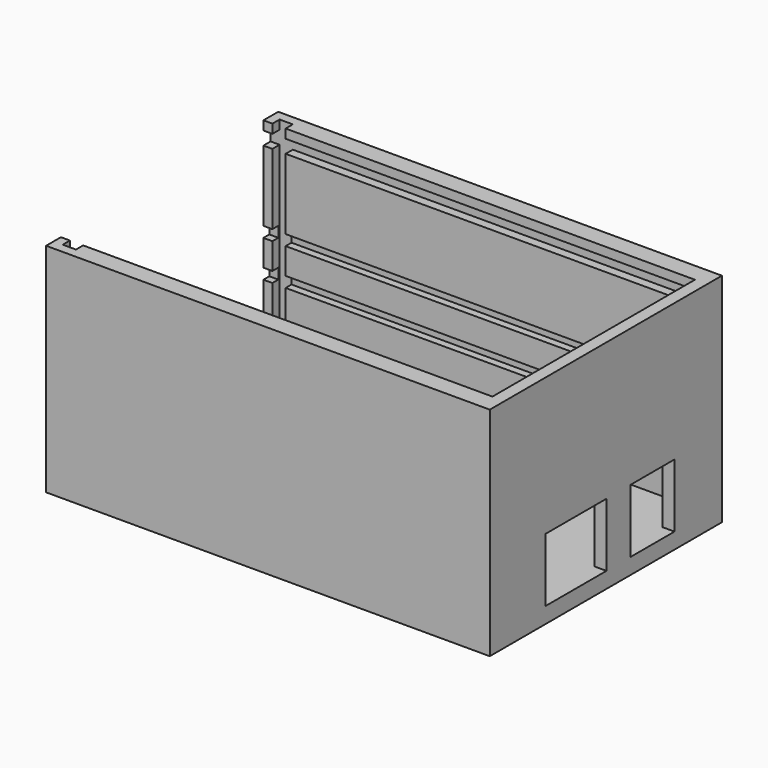
from build123d import *

# Parameters (mm, degrees)
F2_DEPTH  = 41
F1_W      = 1.7
F1_H      = 47.8
F1_W_2    = 77.3
F3_DEPTH  = 3
F1_W_3    = 2.5
F1_H_2    = 1.7
F4_DEPTH  = 1.5
F5_W      = 14.41
F5_H      = 12
F5_W_2    = 10.4
F6_DEPTH  = 3
F7_W      = 1.4
F7_H      = 2
F8_DEPTH  = 81
F9_W      = 1.7
F9_H      = 2.5
F10_DEPTH = 83
F11_W     = 47.8
F11_H     = 2.5
F12_DEPTH = 1.5


with BuildPart() as f2:
    # F1 (on Top) → F2 (new body)
    with BuildSketch(Plane.XY):
        Polygon((-43, 27.4), (-43, 23.9), (-41.3, 23.9), (-41.3, 25.6), (-38.8, 25.6), (-38.8, 23.9), (38.5, 23.9), (38.5, -23.9), (-38.8, -23.9), (-38.8, -25.6), (-41.3, -25.6), (-41.3, -23.9), (-43, -23.9), (-43, -27.4), (40.8, -27.4), (40.8, 27.4), align=None)
    extrude(amount=F2_DEPTH)

    # F1 (on Top) → F3 (join)
    with BuildSketch(Plane.XY):
        with Locations((-42.15, 0)):
            Rectangle(F1_W, F1_H)
        with Locations((-0.15, 0)):
            Rectangle(F1_W_2, F1_H)
    extrude(amount=F3_DEPTH)

    # F1 (on Top) → F4 (join)
    with BuildSketch(Plane.XY):
        with Locations((-40.05, -24.75)):
            Rectangle(F1_W_3, F1_H_2)
        with Locations((-40.05, 0)):
            Rectangle(F1_W_3, F1_H)
        with Locations((-40.05, 24.75)):
            Rectangle(F1_W_3, F1_H_2)
    extrude(amount=F4_DEPTH)

    # F5 (on face) → F6 (cut)
    with BuildSketch(Plane.YZ.offset(40.8)):
        with Locations((-7.065, 9)):
            Rectangle(F5_W, F5_H)
        with Locations((11, 9)):
            Rectangle(F5_W_2, F5_H)
    extrude(amount=-F6_DEPTH, mode=Mode.SUBTRACT)

    # F7 (on face) → F8 (cut)
    with BuildSketch(Plane(origin=(-43, 0, 0), x_dir=(0, -1, 0), z_dir=(-1, 0, 0))):
        with Locations((-24.6, 15.5)):
            Rectangle(F7_W, F7_H)
        with Locations((-24.6, 22.45)):
            Rectangle(F7_W, F7_H)
        with Locations((24.6, 15.5)):
            Rectangle(F7_W, F7_H)
        with Locations((24.6, 22.45)):
            Rectangle(F7_W, F7_H)
    extrude(amount=-F8_DEPTH, mode=Mode.SUBTRACT)

    # F9 (on face) → F10 (cut)
    with BuildSketch(Plane(origin=(-43, 0, 0), x_dir=(0, -1, 0), z_dir=(-1, 0, 0))):
        with Locations((-24.75, 38.05)):
            Rectangle(F9_W, F9_H)
        with Locations((24.75, 38.05)):
            Rectangle(F9_W, F9_H)
    extrude(amount=-F10_DEPTH, mode=Mode.SUBTRACT)

    # F11 (on face) → F12 (cut)
    with BuildSketch(Plane(origin=(38.5, 0, 0), x_dir=(0, -1, 0), z_dir=(-1, 0, 0))):
        with Locations((0, 38.05)):
            Rectangle(F11_W, F11_H)
    extrude(amount=-F12_DEPTH, mode=Mode.SUBTRACT)


solid = f2.part
